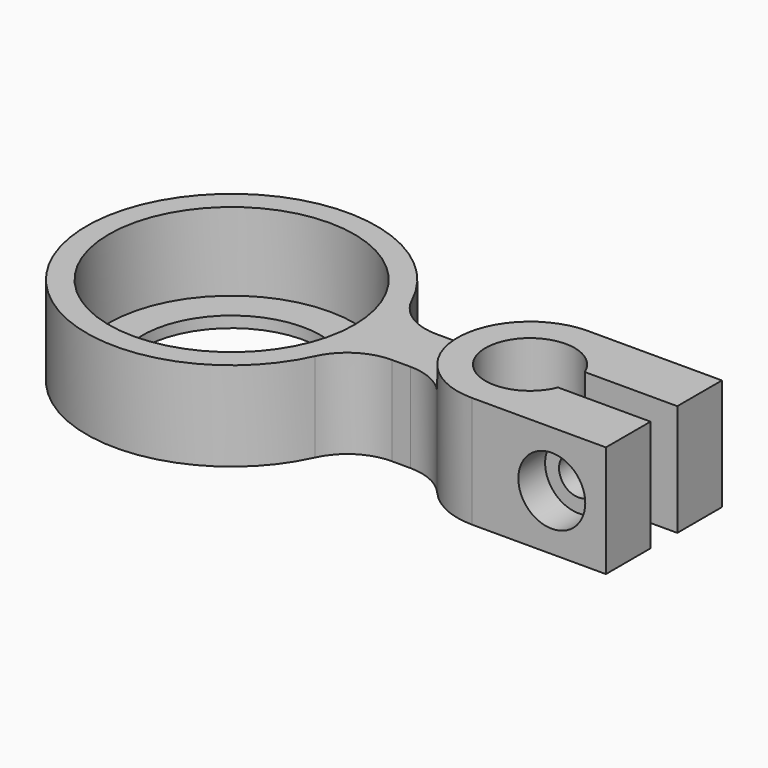
from build123d import *

# Parameters (mm, degrees)
F0_R         = 8
F1_DEPTH     = 10
F2_R         = 11
F3_DEPTH     = 9
F5_DEPTH     = 2
F7_DEPTH     = 3
F8_R         = 1.75
F9_DEPTH     = 19.501
F10_R        = 3
F11_DEPTH    = 3
F12_T1_DEPTH = 8


# Not quite as in the source:
# - a fillet or chamfer that OpenCascade refuses, or shapes differently, is made with other operations: its cross-section is extruded or revolved along the edge and cut away or added


with BuildPart() as f1:
    # F0 (on Top) → F1 (new body)
    with BuildSketch(Plane.XY):
        with BuildLine():
            ThreePointArc((3.7080992435, -1.5), (-4, 0), (3.7080992435, 1.5))
            Line((3.7080992435, 1.5), (12, 1.5))
            Line((12, 1.5), (12, 6.5))
            Line((12, 6.5), (0, 6.5))
            ThreePointArc((0, 6.5), (-3.6055512755, 5.4083269132), (-6, 2.5))
            Line((-6, 2.5), (-13.9926491778, 2.5))
            ThreePointArc((-13.9926491778, 2.5), (-39.75, 0), (-13.9926491778, -2.5))
            Line((-13.9926491778, -2.5), (-6, -2.5))
            ThreePointArc((-6, -2.5), (-3.6055512755, -5.4083269132), (0, -6.5))
            Line((0, -6.5), (12, -6.5))
            Line((12, -6.5), (12, -1.5))
            Line((12, -1.5), (3.7080992435, -1.5))
        make_face()
        with Locations((-26.75, 0)):
            Circle(F0_R, mode=Mode.SUBTRACT)
    extrude(amount=F1_DEPTH)

    # F2 (on face) → F3 (cut)
    with BuildSketch(Plane.XY.offset(10)):
        with Locations((-26.75, 0)):
            Circle(F2_R)
    extrude(amount=-F3_DEPTH, mode=Mode.SUBTRACT)

    # F4 (on face) → F5 (cut)
    with BuildSketch(Plane.XY.offset(10)):
        with BuildLine():
            Line((-6, 2.5), (-13.9926491778, 2.5))
            ThreePointArc((-13.9926491778, 2.5), (-39.75, 0), (-13.9926491778, -2.5))
            Line((-13.9926491778, -2.5), (-6, -2.5))
            ThreePointArc((-6, -2.5), (-6.5, 0), (-6, 2.5))
        make_face()
    extrude(amount=-F5_DEPTH, mode=Mode.SUBTRACT)

    # F6 (on face) → F7 (cut)
    with BuildSketch(Plane(origin=(0, 6.5, 0), x_dir=(-1, 0, 0), z_dir=(0, 1, 0))):
        Polygon((-10, 6.6454482672), (-10, 3.3545517328), (-7.15, 1.7091034656), (-4.3, 3.3545517328), (-4.3, 6.6454482672), (-7.15, 8.2908965344), align=None)
    extrude(amount=-F7_DEPTH, mode=Mode.SUBTRACT)

    # F8 (on face) → F9 (cut, through all)
    with BuildSketch(Plane(origin=(0, 6.5, 0), x_dir=(-1, 0, 0), z_dir=(0, 1, 0))):
        with Locations((-7.15, 5)):
            Circle(F8_R)
    extrude(amount=-F9_DEPTH, mode=Mode.SUBTRACT)

    # F10 (on face) → F11 (cut)
    with BuildSketch(Plane.XZ.offset(6.5)):
        with Locations((7.15, 5)):
            Circle(F10_R)
    extrude(amount=-F11_DEPTH, mode=Mode.SUBTRACT)

    # F12: fillet of radius 5 on 4 edges, made by hand

    # F12_s2 → F12_t1 (join)
    with BuildSketch(Plane.XY):
        with BuildLine():
            ThreePointArc((-8.7177978871, -2.5), (-6.6326537465, -2.9555337043), (-4.9274509797, -4.2391304348))
            ThreePointArc((-4.9274509797, -4.2391304348), (-5.5324894844, -3.4119730516), (-6, -2.5))
            Line((-6, -2.5), (-8.7177978871, -2.5))
        make_face()
        with BuildLine():
            ThreePointArc((-14.9322285425, -5.4166666667), (-13.0872404524, -3.2918729423), (-10.386931828, -2.5))
            Line((-10.386931828, -2.5), (-13.9926491778, -2.5))
            ThreePointArc((-13.9926491778, -2.5), (-14.3762012754, -3.9861140379), (-14.9322285425, -5.4166666667))
        make_face()
        with BuildLine():
            ThreePointArc((-10.386931828, 2.5), (-13.0872404524, 3.2918729423), (-14.9322285425, 5.4166666667))
            ThreePointArc((-14.9322285425, 5.4166666667), (-14.3762012754, 3.9861140379), (-13.9926491778, 2.5))
            Line((-13.9926491778, 2.5), (-10.386931828, 2.5))
        make_face()
        with BuildLine():
            ThreePointArc((-4.9274509797, 4.2391304348), (-6.6326537465, 2.9555337043), (-8.7177978871, 2.5))
            Line((-8.7177978871, 2.5), (-6, 2.5))
            ThreePointArc((-6, 2.5), (-5.5324894844, 3.4119730516), (-4.9274509797, 4.2391304348))
        make_face()
    extrude(amount=F12_T1_DEPTH)


solid = f1.part
